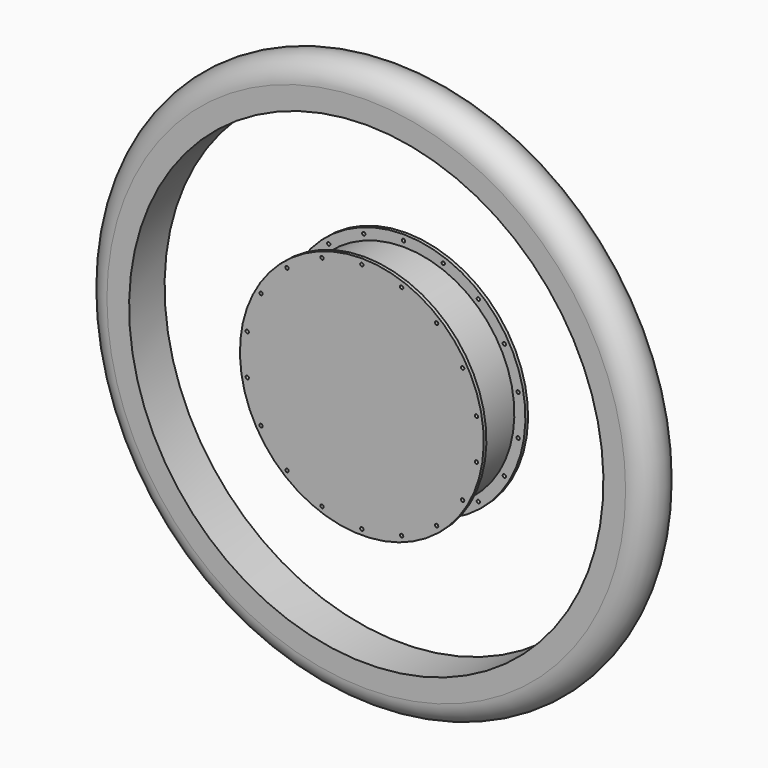
from build123d import *

# Parameters (mm, degrees)
F1_W            = 3
F1_H            = 10
F5_R            = 1.5
F6_DEPTH        = 50.001
F6_COPIES_COUNT = 18


# Not quite as in the source:
# - a pattern or mirror of a feature is missing from the dataset's text; its kind, count and spacing are read off the source's solid


with BuildPart() as f2:
    # F1 (on Right) → F2 (revolve)
    with BuildSketch(Plane.YZ):
        Polygon((25, 0), (25, 100), (22, 100), (-22, 100), (-25, 100), (-25, 0), align=None)
        with Locations((23.5, 105)):
            Rectangle(F1_W, F1_H)
        with Locations((-23.5, 105)):
            Rectangle(F1_W, F1_H)
    revolve(axis=Axis((0, 50.7838092744, 0), (0, 1, 0)))

    # F5 (on face) → F6 (cut, through all)
    with BuildSketch(Plane.XZ.offset(25)):
        with Locations((0, 105)):
            Circle(F5_R)
    f6 = extrude(amount=-F6_DEPTH, mode=Mode.SUBTRACT)

    # F6_copies: F6 ×18 about axis
    f6_copies_axis = Axis((0, 0, 0), (0, 1, 0))
    for i in range(1, F6_COPIES_COUNT):
        add(f6.rotate(f6_copies_axis, i * 360 / F6_COPIES_COUNT), mode=Mode.SUBTRACT)


with BuildPart() as f4:
    # F3 (on Right) → F4 (revolve)
    with BuildSketch(Plane.YZ):
        with BuildLine():
            Line((-20, 214), (20, 214))
            Line((20, 214), (20, 234))
            ThreePointArc((20, 234), (0, 254), (-20, 234))
            Line((-20, 234), (-20, 214))
        make_face()
    revolve(axis=Axis((0, 50.7838092744, 0), (0, 1, 0)))


solid = Compound([f2.part, f4.part])
